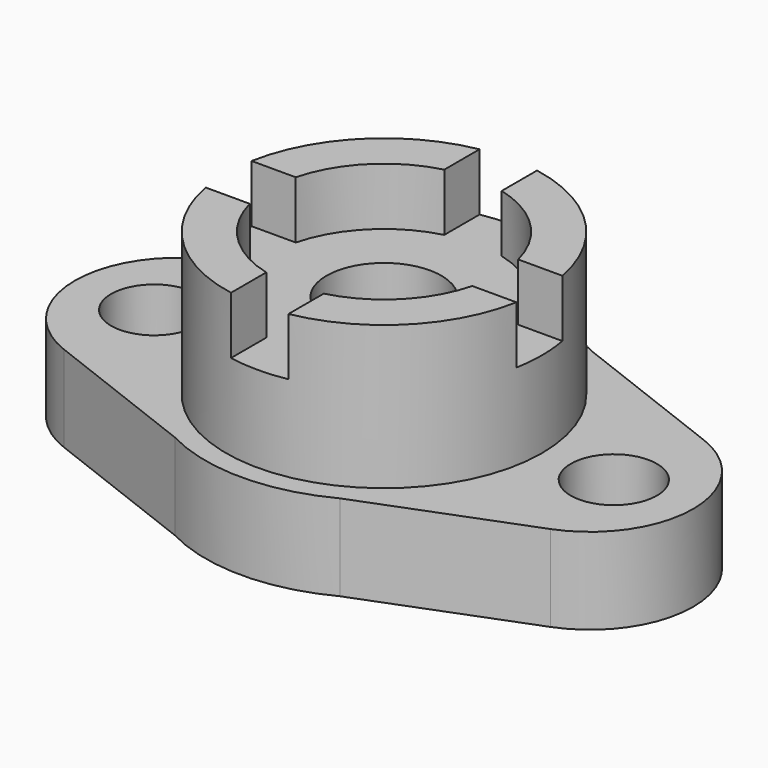
from build123d import *

# Parameters (mm, degrees)
F1_DEPTH = 19.05
F2_DEPTH = 38.1
F3_R     = 34.925
F3_R_2   = 12.7
F4_DEPTH = 12.7
F6_DEPTH = 12.7
F0_R     = 9.525
F7_DEPTH = 19.05
F8_DEPTH = 103.378
F9_DEPTH = 38.1


# Not quite as in the source:
# - a feature names something its author has since deleted; it is built from what else it names


with BuildPart() as f1:
    # F0 (on Top) → F1 (new body)
    with BuildSketch(Plane.XY):
        with BuildLine():
            ThreePointArc((-34.925, 0), (0, -34.925), (34.925, 0))
            Line((34.925, 0), (25.4, 0))
            ThreePointArc((25.4, 0), (0, -25.4), (-25.4, 0))
            Line((-25.4, 0), (-34.925, 0))
        make_face()
        with BuildLine():
            Line((25.4, 0), (34.925, 0))
            ThreePointArc((34.925, 0), (0, 34.925), (-34.925, 0))
            Line((-34.925, 0), (-25.4, 0))
            ThreePointArc((-25.4, 0), (0, 25.4), (25.4, 0))
        make_face()
    extrude(amount=F1_DEPTH)

    # F0 (on Top) → F2 (join)
    with BuildSketch(Plane.XY):
        with BuildLine():
            ThreePointArc((-34.925, 0), (0, -34.925), (34.925, 0))
            Line((34.925, 0), (25.4, 0))
            ThreePointArc((25.4, 0), (0, -25.4), (-25.4, 0))
            Line((-25.4, 0), (-34.925, 0))
        make_face()
        with BuildLine():
            Line((25.4, 0), (34.925, 0))
            ThreePointArc((34.925, 0), (0, 34.925), (-34.925, 0))
            Line((-34.925, 0), (-25.4, 0))
            ThreePointArc((-25.4, 0), (0, 25.4), (25.4, 0))
        make_face()
        with BuildLine():
            ThreePointArc((-25.4, 0), (0, -25.4), (25.4, 0))
            Line((25.4, 0), (12.7, 0))
            ThreePointArc((12.7, 0), (0, -12.7), (-12.7, 0))
            Line((-12.7, 0), (-25.4, 0))
        make_face()
        with BuildLine():
            Line((12.7, 0), (25.4, 0))
            ThreePointArc((25.4, 0), (0, 25.4), (-25.4, 0))
            Line((-25.4, 0), (-12.7, 0))
            ThreePointArc((-12.7, 0), (0, 12.7), (12.7, 0))
        make_face()
    extrude(amount=F2_DEPTH)

    # F3 (on face) → F4 (join)
    with BuildSketch(Plane.XY.offset(38.1)):
        Circle(F3_R)
        Circle(F3_R_2, mode=Mode.SUBTRACT)
    extrude(amount=F4_DEPTH)

    # F5 (on face) → F6 (cut)
    with BuildSketch(Plane.XY.offset(50.8)):
        with BuildLine():
            ThreePointArc((-24.5934442484, -6.35), (-25.4, 0), (-24.5934442484, 6.35))
            Line((-24.5934442484, 6.35), (-34.3428758988, 6.35))
            ThreePointArc((-34.3428758988, 6.35), (-34.925, 0), (-34.3428758988, -6.35))
            Line((-34.3428758988, -6.35), (-24.5934442484, -6.35))
        make_face()
        with BuildLine():
            Line((6.35, -34.3428758988), (6.35, -24.5934442484))
            ThreePointArc((6.35, -24.5934442484), (0, -25.4), (-6.35, -24.5934442484))
            Line((-6.35, -24.5934442484), (-6.35, -34.3428758988))
            ThreePointArc((-6.35, -34.3428758988), (0, -34.925), (6.35, -34.3428758988))
        make_face()
        with BuildLine():
            Line((34.3428758988, 6.35), (24.5934442484, 6.35))
            ThreePointArc((24.5934442484, 6.35), (25.1975542852, 3.2005090291), (25.4, 0))
            ThreePointArc((25.4, 0), (25.1975542852, -3.2005090291), (24.5934442484, -6.35))
            Line((24.5934442484, -6.35), (34.3428758988, -6.35))
            ThreePointArc((34.3428758988, -6.35), (34.7791644937, -3.1883133656), (34.925, 0))
            ThreePointArc((34.925, 0), (34.7791644937, 3.1883133656), (34.3428758988, 6.35))
        make_face()
        with BuildLine():
            ThreePointArc((-6.35, 24.5934442484), (0, 25.4), (6.35, 24.5934442484))
            Line((6.35, 24.5934442484), (6.35, 34.3428758988))
            ThreePointArc((6.35, 34.3428758988), (0, 34.925), (-6.35, 34.3428758988))
            Line((-6.35, 34.3428758988), (-6.35, 24.5934442484))
        make_face()
    extrude(amount=-F6_DEPTH, mode=Mode.SUBTRACT)

    # F0 (on Top) → F7 (join)
    with BuildSketch(Plane.XY):
        with BuildLine():
            Line((53.7687589873, 21.2442149995), (18.2328532376, 34.9850083733))
            ThreePointArc((18.2328532376, 34.9850083733), (0, 39.4510804423), (-18.2328532376, 34.9850083733))
            Line((-18.2328532376, 34.9850083733), (-53.7687589873, 21.2442149995))
            ThreePointArc((-53.7687589873, 21.2442149995), (-68.3312757395, 0), (-53.7687589873, -21.2442149995))
            Line((-53.7687589873, -21.2442149995), (-18.2328532376, -34.9850083733))
            ThreePointArc((-18.2328532376, -34.9850083733), (0, -39.4510804423), (18.2328532376, -34.9850083733))
            Line((18.2328532376, -34.9850083733), (53.7687589873, -21.2442149995))
            ThreePointArc((53.7687589873, -21.2442149995), (68.3312757395, 0), (53.7687589873, 21.2442149995))
        make_face()
        with Locations((-50.8, 0)):
            Circle(F0_R, mode=Mode.SUBTRACT)
        with BuildLine():
            ThreePointArc((-34.925, 0), (0, 34.925), (34.925, 0))
            ThreePointArc((34.925, 0), (0, -34.925), (-34.925, 0))
        make_face(mode=Mode.SUBTRACT)
        with BuildLine():
            ThreePointArc((60.325, 0), (50.8, -9.525), (41.275, 0))
            ThreePointArc((41.275, 0), (50.8, 9.525), (60.325, 0))
        make_face(mode=Mode.SUBTRACT)
    extrude(amount=F7_DEPTH)

    # F5 (on face) → F8 (cut)
    with BuildSketch(Plane.XY.offset(50.8)):
        with BuildLine():
            Line((6.35, 6.35), (6.35, 0))
            Line((6.35, 0), (6.35, -6.35))
            Line((6.35, -6.35), (24.5934442484, -6.35))
            ThreePointArc((24.5934442484, -6.35), (25.1975542852, -3.2005090291), (25.4, 0))
            ThreePointArc((25.4, 0), (25.1975542852, 3.2005090291), (24.5934442484, 6.35))
            Line((24.5934442484, 6.35), (6.35, 6.35))
        make_face()
        with BuildLine():
            Line((-6.35, -6.35), (-6.35, 0))
            Line((-6.35, 0), (-6.35, 6.35))
            Line((-6.35, 6.35), (-24.5934442484, 6.35))
            ThreePointArc((-24.5934442484, 6.35), (-25.4, 0), (-24.5934442484, -6.35))
            Line((-24.5934442484, -6.35), (-6.35, -6.35))
        make_face()
        with BuildLine():
            Line((-6.35, 6.35), (0, 6.35))
            Line((0, 6.35), (6.35, 6.35))
            Line((6.35, 6.35), (6.35, 24.5934442484))
            ThreePointArc((6.35, 24.5934442484), (0, 25.4), (-6.35, 24.5934442484))
            Line((-6.35, 24.5934442484), (-6.35, 6.35))
        make_face()
        with BuildLine():
            Line((6.35, -6.35), (0, -6.35))
            Line((0, -6.35), (-6.35, -6.35))
            Line((-6.35, -6.35), (-6.35, -24.5934442484))
            ThreePointArc((-6.35, -24.5934442484), (0, -25.4), (6.35, -24.5934442484))
            Line((6.35, -24.5934442484), (6.35, -6.35))
        make_face()
        with BuildLine():
            Line((6.35, 24.5934442484), (6.35, 6.35))
            Line((6.35, 6.35), (24.5934442484, 6.35))
            ThreePointArc((24.5934442484, 6.35), (17.9605122421, 17.9605122421), (6.35, 24.5934442484))
        make_face()
        with BuildLine():
            Line((24.5934442484, -6.35), (6.35, -6.35))
            Line((6.35, -6.35), (6.35, -24.5934442484))
            ThreePointArc((6.35, -24.5934442484), (17.9605122421, -17.9605122421), (24.5934442484, -6.35))
        make_face()
        with BuildLine():
            Line((-24.5934442484, 6.35), (-6.35, 6.35))
            Line((-6.35, 6.35), (-6.35, 24.5934442484))
            ThreePointArc((-6.35, 24.5934442484), (-17.9605122421, 17.9605122421), (-24.5934442484, 6.35))
        make_face()
        with BuildLine():
            Line((-6.35, -24.5934442484), (-6.35, -6.35))
            Line((-6.35, -6.35), (-24.5934442484, -6.35))
            ThreePointArc((-24.5934442484, -6.35), (-17.9605122421, -17.9605122421), (-6.35, -24.5934442484))
        make_face()
    extrude(amount=-F8_DEPTH, mode=Mode.SUBTRACT)

    # F0 (on Top) → F9 (join)
    with BuildSketch(Plane.XY):
        with BuildLine():
            ThreePointArc((-25.4, 0), (0, -25.4), (25.4, 0))
            Line((25.4, 0), (12.7, 0))
            ThreePointArc((12.7, 0), (0, -12.7), (-12.7, 0))
            Line((-12.7, 0), (-25.4, 0))
        make_face()
        with BuildLine():
            Line((12.7, 0), (25.4, 0))
            ThreePointArc((25.4, 0), (0, 25.4), (-25.4, 0))
            Line((-25.4, 0), (-12.7, 0))
            ThreePointArc((-12.7, 0), (0, 12.7), (12.7, 0))
        make_face()
    extrude(amount=F9_DEPTH)


solid = f1.part
